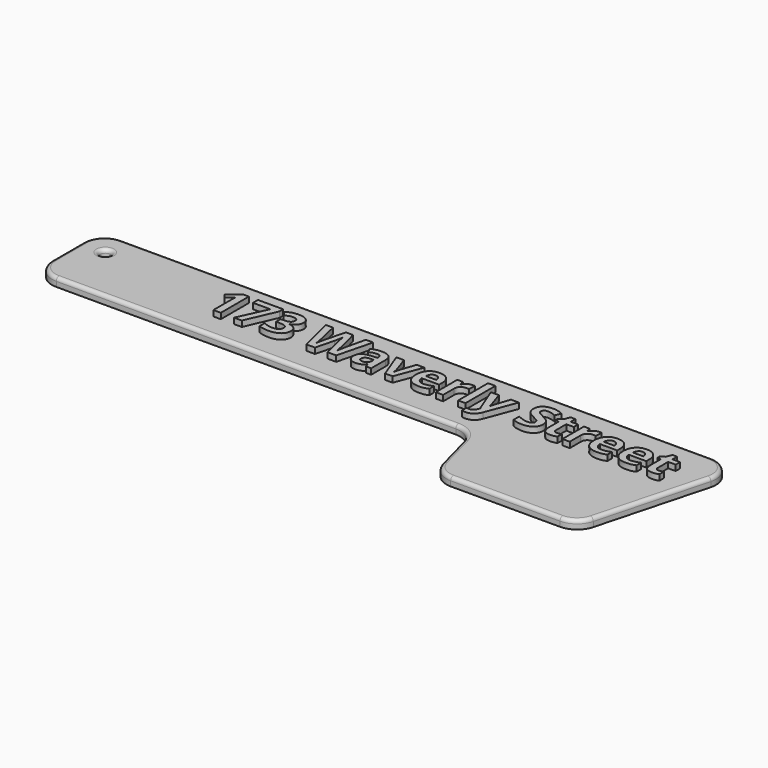
from build123d import *

# Parameters (mm, degrees)
F0_R         = 1.905
F1_DEPTH     = 3.048
F2_R         = 7.62
F3_R         = 1.27
F4_TEXT_SIZE = 17.605091721
F5_DEPTH     = 2.032


# Not quite as in the source:
# - Text() gives the source's letters only with a copy of the font that has no kerning and outlines rounded to 1/6400 em; it was checked with that copy


with BuildPart() as f1:
    # F0 (on Top) → F1 (new body)
    with BuildSketch(Plane.XY):
        Polygon((219.71, 8.89), (-8.89, 8.89), (-8.89, -20.32), (147.4713851136, -20.32), (154.2772946013, -45.72), (205.0772946013, -45.72), align=None)
        Circle(F0_R, mode=Mode.SUBTRACT)
    extrude(amount=F1_DEPTH)

    # F2
    f2_edges = [f1.edges().sort_by_distance(p)[0] for p in [
        (154.277295, -45.72, 1.524),
        (205.077295, -45.72, 1.524),
        (219.71, 8.89, 1.524),
        (-8.89, -20.32, 1.524),
        (-8.89, 8.89, 1.524),
        (147.471385, -20.32, 1.524),
    ]]
    fillet(f2_edges, radius=F2_R)

    # F3
    f3_edges = [f1.edges().sort_by_distance(p)[0] for p in [
        (104.254711, 8.89, 3.048),
        (215.824775, 5.908762, 3.048),
        (-6.658154, 6.658154, 3.048),
        (211.865198, -20.387201, 3.048),
        (-8.89, -5.715, 3.048),
        (203.869025, -44.145352, 3.048),
        (-6.658154, -18.088154, 3.048),
        (179.677295, -45.72, 3.048),
        (70.177177, -20.32, 3.048),
        (155.485564, -44.145352, 3.048),
        (146.263116, -21.894648, 3.048),
        (150.87434, -33.02, 3.048),
        (-1.905, 0, 3.048),
    ]]
    fillet(f3_edges, radius=F3_R)

    # F4 (on face) → F5 (join)
    with BuildSketch(Plane.XY.offset(3.048)):
        with Locations((43.18, -11.43)):
            Text('173 Waverly Street', F4_TEXT_SIZE, font='Open Sans', font_style=FontStyle.BOLD, text_align=(TextAlign.LEFT, TextAlign.BOTTOM))
    extrude(amount=F5_DEPTH)


solid = f1.part
